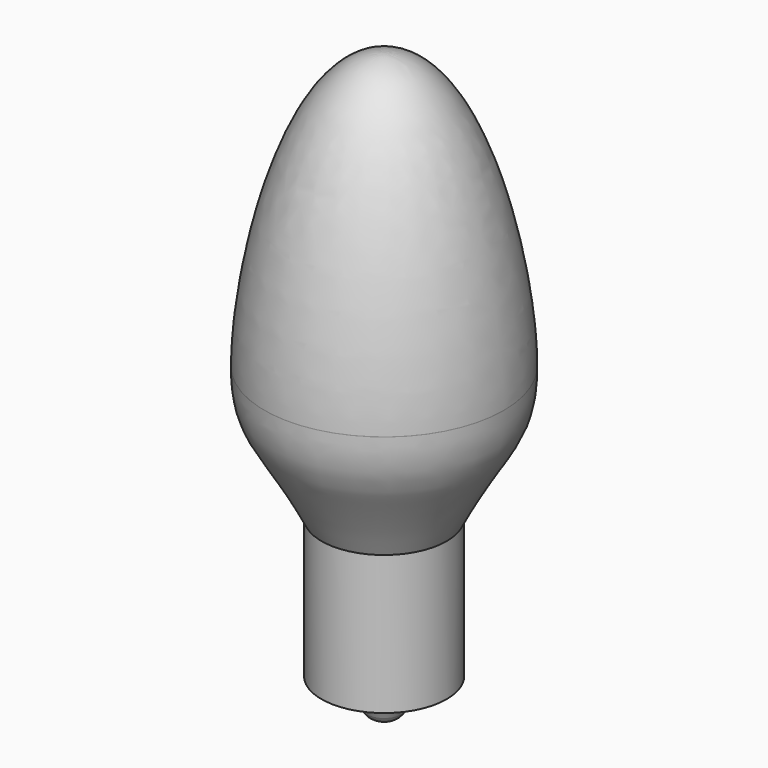
from build123d import *


# Not quite as in the source:
# - ends of sketch curves that miss each other by under 0.0002 mm in the source are joined


with BuildPart() as f2:
    # F0 (on Front) → F2 (revolve)
    with BuildSketch(Plane.XZ):
        with BuildLine():
            Line((1.5679514959, -15.2930365572), (2.8448, -12.7))
            Line((2.8448, -12.7), (5.715, -12.7))
            Line((5.715, -12.7), (5.715, 0))
            Line((5.715, 0), (0, 0))
            Line((0, 0), (0, -16.002))
            Line((0, -16.002), (0.4285929126, -16.002))
            ThreePointArc((0.4285929126, -16.002), (1.0995562396, -15.8102894852), (1.5679514959, -15.2930365572))
        make_face()
    revolve(axis=Axis((0, 0, 12.4274427071), (0, 0, -1)))


with BuildPart() as f3_1:
    # F3: copy of F2
    add(f2.part)


with BuildPart() as f2_1:
    add(f2.part)

    # F0 (on Front) → F5 (revolve)
    with BuildSketch(Plane.XZ):
        with BuildLine():
            Line((0, 0), (5.715, 0))
            add(Edge.make_bspline(
                [(5.715, 0), (9.213257581, 7.0497766137), (10.9194947638, 7.0893163742), (10.922, 12.192)],
                knots=[0, 0, 0, 0, 0.4101662252, 0.4101662252, 0.4101662252, 0.4101662252], degree=3))
            Line((10.922, 12.192), (10.922, 12.2032626975))
            add(Edge.make_bspline(
                [(10.922, 12.2032626975), (10.9220027628, 19.5480467726), (7.4021908993, 37.338), (0, 37.338)],
                knots=[0.4104677797, 0.4104677797, 0.4104677797, 0.4104677797, 1, 1, 1, 1], degree=3))
            Line((0, 37.338), (0, 0))
        make_face()
    revolve(axis=Axis((0, 0, 12.4274427071), (0, 0, -1)))


with BuildPart() as f6_1:
    # F6: copy of F2
    add(f2_1.part)


solid = f2_1.part
